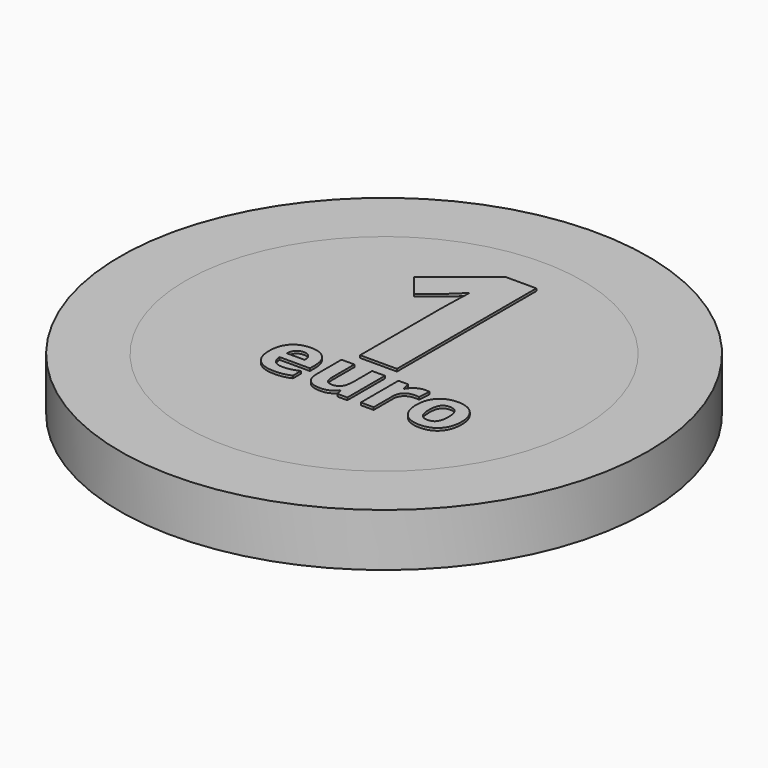
from build123d import *

# Parameters (mm, degrees)
F0_R           = 11.625
F0_R_2         = 8.7396935436
F1_DEPTH       = 2.33
F0_TEXT_SIZE   = 10.7492641999
F0_TEXT_SIZE_2 = 3.7975795244
F2_DEPTH       = 2.33
F3_DEPTH       = 2.4384


# Not quite as in the source:
# - Text() gives the source's letters only with a copy of the font that has no kerning and outlines rounded to 1/6400 em; it was checked with that copy


with BuildPart() as f1:
    # F0 (on Top) → F1 (new body)
    with BuildSketch(Plane.XY):
        Circle(F0_R)
        Circle(F0_R_2, mode=Mode.SUBTRACT)
    extrude(amount=F1_DEPTH)


with BuildPart() as f2:
    # F0 (on Top) → F2 (new body)
    with BuildSketch(Plane.XY):
        Circle(F0_R_2)
        with BuildLine():
            add(Edge.make_bspline(
                [(-1.6260833649, -3.4872782475), (-1.7946009563, -3.5234739273), (-2.0378833946, -3.5234739273)],
                knots=[0, 0, 0, 1, 1, 1], degree=2))
            add(Edge.make_bspline(
                [(-2.0378833946, -3.5234739273), (-2.5380958225, -3.5234739273), (-2.8199474279, -3.2469626682)],
                knots=[0, 0, 0, 1, 1, 1], degree=2))
            add(Edge.make_bspline(
                [(-2.8199474279, -3.2469626682), (-3.1017990332, -2.9704514091), (-3.1017990332, -2.4643052631)],
                knots=[0, 0, 0, 1, 1, 1], degree=2))
            add(Edge.make_bspline(
                [(-3.1017990332, -2.4643052631), (-3.1017990332, -1.9433248221), (-2.8413088127, -1.6588030437)],
                knots=[0, 0, 0, 1, 1, 1], degree=2))
            add(Edge.make_bspline(
                [(-2.8413088127, -1.6588030437), (-2.5808185922, -1.3742812652), (-2.1209554466, -1.3742812652)],
                knots=[0, 0, 0, 1, 1, 1], degree=2))
            add(Edge.make_bspline(
                [(-2.1209554466, -1.3742812652), (-1.6818603141, -1.3742812652), (-1.4370944464, -1.6243874792)],
                knots=[0, 0, 0, 1, 1, 1], degree=2))
            add(Edge.make_bspline(
                [(-1.4370944464, -1.6243874792), (-1.1923285786, -1.8744936932), (-1.1923285786, -2.3159623129)],
                knots=[0, 0, 0, 1, 1, 1], degree=2))
            Line((-1.1923285786, -2.3159623129), (-1.1923285786, -2.5906934566))
            Line((-1.1923285786, -2.5906934566), (-2.5291952455, -2.5906934566))
            add(Edge.make_bspline(
                [(-2.5291952455, -2.5906934566), (-2.5197012967, -2.8316024077), (-2.3861926416, -2.9668911783)],
                knots=[0, 0, 0, 1, 1, 1], degree=2))
            add(Edge.make_bspline(
                [(-2.3861926416, -2.9668911783), (-2.2526839864, -3.1021799488), (-2.0117750353, -3.1021799488)],
                knots=[0, 0, 0, 1, 1, 1], degree=2))
            add(Edge.make_bspline(
                [(-2.0117750353, -3.1021799488), (-1.8242695463, -3.1021799488), (-1.6575320703, -3.0633140959)],
                knots=[0, 0, 0, 1, 1, 1], degree=2))
            add(Edge.make_bspline(
                [(-1.6575320703, -3.0633140959), (-1.4907945943, -3.0244482429), (-1.3092228233, -2.9390027036)],
                knots=[0, 0, 0, 1, 1, 1], degree=2))
            Line((-1.3092228233, -2.9390027036), (-1.3092228233, -3.3769110925))
            add(Edge.make_bspline(
                [(-1.3092228233, -3.3769110925), (-1.4575657735, -3.4510825676), (-1.6260833649, -3.4872782475)],
                knots=[0, 0, 0, 1, 1, 1], degree=2))
        make_face(mode=Mode.SUBTRACT)
        with BuildLine():
            Line((1.1698845599, -3.4860915039), (0.7361297736, -3.4860915039))
            Line((0.7361297736, -3.4860915039), (0.6601781832, -3.220854309))
            Line((0.6601781832, -3.220854309), (0.6305095931, -3.220854309))
            add(Edge.make_bspline(
                [(0.6305095931, -3.220854309), (0.5397237076, -3.3656370283), (0.3726895457, -3.4445554778)],
                knots=[0, 0, 0, 1, 1, 1], degree=2))
            add(Edge.make_bspline(
                [(0.3726895457, -3.4445554778), (0.2056553838, -3.5234739273), (-0.0073650926, -3.5234739273)],
                knots=[0, 0, 0, 1, 1, 1], degree=2))
            add(Edge.make_bspline(
                [(-0.0073650926, -3.5234739273), (-0.3728821218, -3.5234739273), (-0.5583108096, -3.3276612331)],
                knots=[0, 0, 0, 1, 1, 1], degree=2))
            add(Edge.make_bspline(
                [(-0.5583108096, -3.3276612331), (-0.7437394973, -3.1318485389), (-0.7437394973, -2.7645513942)],
                knots=[0, 0, 0, 1, 1, 1], degree=2))
            Line((-0.7437394973, -2.7645513942), (-0.7437394973, -1.4128504323))
            Line((-0.7437394973, -1.4128504323), (-0.1782561712, -1.4128504323))
            Line((-0.1782561712, -1.4128504323), (-0.1782561712, -2.6239222775))
            add(Edge.make_bspline(
                [(-0.1782561712, -2.6239222775), (-0.1782561712, -2.8482168181), (-0.098447664, -2.9603640885)],
                knots=[0, 0, 0, 1, 1, 1], degree=2))
            add(Edge.make_bspline(
                [(-0.098447664, -2.9603640885), (-0.0186391568, -3.0725113588), (0.1558121526, -3.0725113588)],
                knots=[0, 0, 0, 1, 1, 1], degree=2))
            add(Edge.make_bspline(
                [(0.1558121526, -3.0725113588), (0.3931608728, -3.0725113588), (0.4987810534, -2.914081088)],
                knots=[0, 0, 0, 1, 1, 1], degree=2))
            add(Edge.make_bspline(
                [(0.4987810534, -2.914081088), (0.6044012339, -2.7556508172), (0.6044012339, -2.3883536726)],
                knots=[0, 0, 0, 1, 1, 1], degree=2))
            Line((0.6044012339, -2.3883536726), (0.6044012339, -1.4128504323))
            Line((0.6044012339, -1.4128504323), (1.1698845599, -1.4128504323))
            Line((1.1698845599, -1.4128504323), (1.1698845599, -3.4860915039))
        make_face(mode=Mode.SUBTRACT)
        with BuildLine():
            add(Edge.make_bspline(
                [(2.5634182338, -1.4807915035), (2.7274855367, -1.3742812652), (2.9203313719, -1.3742812652)],
                knots=[0, 0, 0, 1, 1, 1], degree=2))
            add(Edge.make_bspline(
                [(2.9203313719, -1.3742812652), (3.0354455013, -1.3742812652), (3.1113970918, -1.3908956757)],
                knots=[0, 0, 0, 1, 1, 1], degree=2))
            Line((3.1113970918, -1.3908956757), (3.0686743221, -1.9207766937))
            add(Edge.make_bspline(
                [(3.0686743221, -1.9207766937), (2.9998431932, -1.9023821679), (2.9019368461, -1.9023821679)],
                knots=[0, 0, 0, 1, 1, 1], degree=2))
            add(Edge.make_bspline(
                [(2.9019368461, -1.9023821679), (2.631359305, -1.9023821679), (2.4800494958, -2.0415278551)],
                knots=[0, 0, 0, 1, 1, 1], degree=2))
            add(Edge.make_bspline(
                [(2.4800494958, -2.0415278551), (2.3287396867, -2.1806735424), (2.3287396867, -2.4310764423)],
                knots=[0, 0, 0, 1, 1, 1], degree=2))
            Line((2.3287396867, -2.4310764423), (2.3287396867, -3.4860915039))
            Line((2.3287396867, -3.4860915039), (1.7632563606, -3.4860915039))
            Line((1.7632563606, -3.4860915039), (1.7632563606, -1.4128504323))
            Line((1.7632563606, -1.4128504323), (2.1916708007, -1.4128504323))
            Line((2.1916708007, -1.4128504323), (2.2753362246, -1.7617530511))
            Line((2.2753362246, -1.7617530511), (2.3026313274, -1.7617530511))
            add(Edge.make_bspline(
                [(2.3026313274, -1.7617530511), (2.3993509309, -1.5873017417), (2.5634182338, -1.4807915035)],
                knots=[0, 0, 0, 1, 1, 1], degree=2))
        make_face(mode=Mode.SUBTRACT)
        with BuildLine():
            add(Edge.make_bspline(
                [(5.2493156896, -1.8765704945), (5.3715502806, -2.1195562469), (5.3715502806, -2.4459107373)],
                knots=[0, 0, 0, 1, 1, 1], degree=2))
            add(Edge.make_bspline(
                [(5.3715502806, -2.4459107373), (5.3715502806, -2.9520568833), (5.1045329703, -3.2377654053)],
                knots=[0, 0, 0, 1, 1, 1], degree=2))
            add(Edge.make_bspline(
                [(5.1045329703, -3.2377654053), (4.83751566, -3.5234739273), (4.361038104, -3.5234739273)],
                knots=[0, 0, 0, 1, 1, 1], degree=2))
            add(Edge.make_bspline(
                [(4.361038104, -3.5234739273), (4.0625720883, -3.5234739273), (3.8344206309, -3.3926354453)],
                knots=[0, 0, 0, 1, 1, 1], degree=2))
            add(Edge.make_bspline(
                [(3.8344206309, -3.3926354453), (3.6062691735, -3.2617969632), (3.4840345826, -3.0170310954)],
                knots=[0, 0, 0, 1, 1, 1], degree=2))
            add(Edge.make_bspline(
                [(3.4840345826, -3.0170310954), (3.3617999917, -2.7722652277), (3.3617999917, -2.4459107373)],
                knots=[0, 0, 0, 1, 1, 1], degree=2))
            add(Edge.make_bspline(
                [(3.3617999917, -2.4459107373), (3.3617999917, -1.9379844759), (3.6267405007, -1.6561328706)],
                knots=[0, 0, 0, 1, 1, 1], degree=2))
            add(Edge.make_bspline(
                [(3.6267405007, -1.6561328706), (3.8916810097, -1.3742812652), (4.3723121682, -1.3742812652)],
                knots=[0, 0, 0, 1, 1, 1], degree=2))
            add(Edge.make_bspline(
                [(4.3723121682, -1.3742812652), (4.670778184, -1.3742812652), (4.8989296413, -1.5039330037)],
                knots=[0, 0, 0, 1, 1, 1], degree=2))
            add(Edge.make_bspline(
                [(4.8989296413, -1.5039330037), (5.1270810987, -1.6335847421), (5.2493156896, -1.8765704945)],
                knots=[0, 0, 0, 1, 1, 1], degree=2))
        make_face(mode=Mode.SUBTRACT)
        with BuildLine():
            Line((1.1680996608, 6.9221326488), (1.1680996608, -0.7518342463))
            Line((1.1680996608, -0.7518342463), (-0.4543674044, -0.7518342463))
            Line((-0.4543674044, -0.7518342463), (-0.4543674044, 3.6889555262))
            Line((-0.4543674044, 3.6889555262), (-0.4375716791, 4.4178900048))
            Line((-0.4375716791, 4.4178900048), (-0.4123780911, 5.2156869571))
            add(Edge.make_bspline(
                [(-0.4123780911, 5.2156869571), (-0.8154754986, 4.8125895496), (-0.9733553165, 4.6866216098)],
                knots=[0, 0, 0, 1, 1, 1], degree=2))
            Line((-0.9733553165, 4.6866216098), (-1.8551308954, 3.9778420016))
            Line((-1.8551308954, 3.9778420016), (-2.637811695, 4.9536736422))
            Line((-2.637811695, 4.9536736422), (-0.165480929, 6.9221326488))
            Line((-0.165480929, 6.9221326488), (1.1680996608, 6.9221326488))
        make_face(mode=Mode.SUBTRACT)
        with Locations((-3.2726901118, -0.7518342463)):
            Text('1', F0_TEXT_SIZE, font='Open Sans', font_style=FontStyle.BOLD, text_align=(TextAlign.LEFT, TextAlign.BOTTOM))
        with Locations((-3.2726901118, -3.4860915039)):
            Text('euro', F0_TEXT_SIZE_2, font='Open Sans', font_style=FontStyle.BOLD, text_align=(TextAlign.LEFT, TextAlign.BOTTOM))
        with BuildLine():
            add(Edge.make_bspline(
                [(4.0382438444, -1.9830807327), (3.9379640101, -2.1361706573), (3.9379640101, -2.4459107373)],
                knots=[0, 0, 0, 1, 1, 1], degree=2))
            add(Edge.make_bspline(
                [(3.9379640101, -2.4459107373), (3.9379640101, -2.7538707018), (4.0391339021, -2.9114109149)],
                knots=[0, 0, 0, 1, 1, 1], degree=2))
            add(Edge.make_bspline(
                [(4.0391339021, -2.9114109149), (4.1403037942, -3.068951128), (4.3681585656, -3.068951128)],
                knots=[0, 0, 0, 1, 1, 1], degree=2))
            add(Edge.make_bspline(
                [(4.3681585656, -3.068951128), (4.5948265935, -3.068951128), (4.6939196842, -2.9123009726)],
                knots=[0, 0, 0, 1, 1, 1], degree=2))
            add(Edge.make_bspline(
                [(4.6939196842, -2.9123009726), (4.7930127749, -2.7556508172), (4.7930127749, -2.4459107373)],
                knots=[0, 0, 0, 1, 1, 1], degree=2))
            add(Edge.make_bspline(
                [(4.7930127749, -2.4459107373), (4.7930127749, -2.1379507727), (4.6930296265, -1.9839707904)],
                knots=[0, 0, 0, 1, 1, 1], degree=2))
            add(Edge.make_bspline(
                [(4.6930296265, -1.9839707904), (4.5930464781, -1.8299908082), (4.3645983348, -1.8299908082)],
                knots=[0, 0, 0, 1, 1, 1], degree=2))
            add(Edge.make_bspline(
                [(4.3645983348, -1.8299908082), (4.1385236787, -1.8299908082), (4.0382438444, -1.9830807327)],
                knots=[0, 0, 0, 1, 1, 1], degree=2))
        make_face()
        with BuildLine():
            add(Edge.make_bspline(
                [(-1.8319833797, -1.8905147318), (-1.9376035602, -1.7765873461), (-2.1173952158, -1.7765873461)],
                knots=[0, 0, 0, 1, 1, 1], degree=2))
            add(Edge.make_bspline(
                [(-2.1173952158, -1.7765873461), (-2.2971868714, -1.7765873461), (-2.3992468212, -1.8905147318)],
                knots=[0, 0, 0, 1, 1, 1], degree=2))
            add(Edge.make_bspline(
                [(-2.3992468212, -1.8905147318), (-2.5013067709, -2.0044421176), (-2.5161410659, -2.2139023632)],
                knots=[0, 0, 0, 1, 1, 1], degree=2))
            Line((-2.5161410659, -2.2139023632), (-1.7222095966, -2.2139023632))
            add(Edge.make_bspline(
                [(-1.7222095966, -2.2139023632), (-1.7263631992, -2.0044421176), (-1.8319833797, -1.8905147318)],
                knots=[0, 0, 0, 1, 1, 1], degree=2))
        make_face()
    extrude(amount=F2_DEPTH)

    # F0 (on Top) → F3 (join)
    with BuildSketch(Plane.XY):
        with Locations((-3.2726901118, -0.7518342463)):
            Text('1', F0_TEXT_SIZE, font='Open Sans', font_style=FontStyle.BOLD, text_align=(TextAlign.LEFT, TextAlign.BOTTOM))
        with Locations((-3.2726901118, -3.4860915039)):
            Text('euro', F0_TEXT_SIZE_2, font='Open Sans', font_style=FontStyle.BOLD, text_align=(TextAlign.LEFT, TextAlign.BOTTOM))
    extrude(amount=F3_DEPTH)


solid = Compound([f1.part, f2.part])
